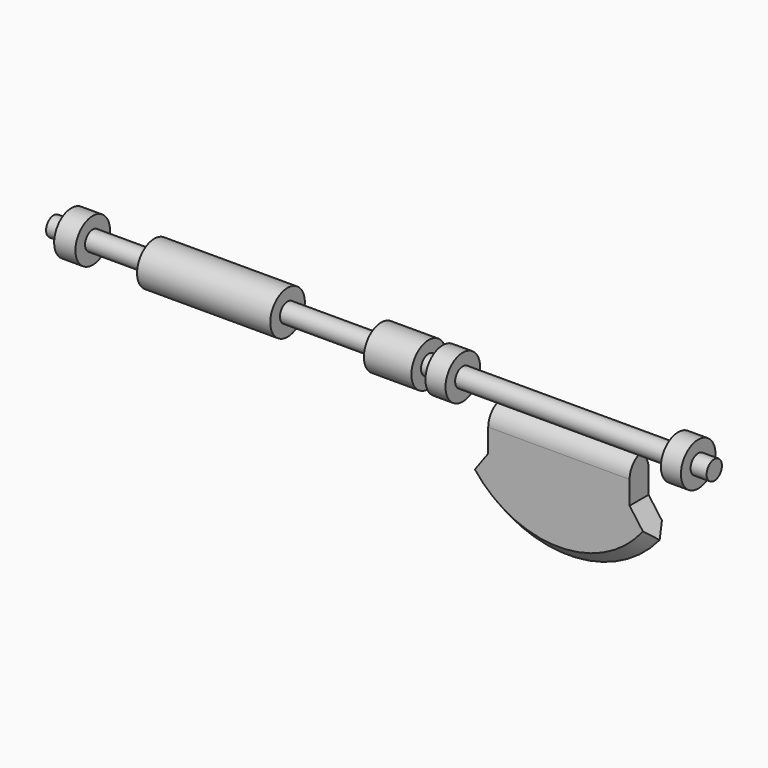
from build123d import *

# Parameters (mm, degrees)
F2_DEPTH    = 3.302
F3_DEPTH    = 3.302
F4_T2_ANGLE = 142.4839860816
F4_T4_ANGLE = 142.4839860816
F5_T1_DEPTH = 64.7221527338


# Not quite as in the source:
# - a fillet or chamfer that OpenCascade refuses, or shapes differently, is made with other operations: its cross-section is extruded or revolved along the edge and cut away or added


with BuildPart() as f1:
    # F0 (on Front) → F1 (revolve)
    with BuildSketch(Plane.XZ):
        Polygon((-57.3470704257, 12.4153448269), (-57.3470704257, 9.7549136262), (126.3579279184, 9.7549136262), (126.3579279184, 12.4153448269), (121.8937337399, 12.4153448269), (121.8937337399, 15.7655160874), (116.3134798408, 15.7655160874), (116.3134798408, 12.4153448269), (56.4188025892, 12.4153448269), (56.4188025892, 15.7655160874), (50.8385524154, 15.7655160874), (50.8385524154, 12.4153448269), (46.9323731959, 12.4153448269), (46.9323731959, 15.7655160874), (33.7257832289, 15.7655160874), (33.7257832289, 12.4153448269), (7.6856887899, 12.4153448269), (7.6856887899, 15.7655160874), (-29.3632764369, 15.7655160874), (-29.3632764369, 12.4153448269), (-46.5082786977, 12.4153448269), (-46.5082786977, 15.7655160874), (-52.420347929, 15.7655160874), (-52.420347929, 12.4153448269), align=None)
    revolve(axis=Axis((34.5054287463, 0, 9.7549136262), (1, 0, 0)))


with BuildPart() as f2:
    # F0 (on Front) → F2 (new body)
    with BuildSketch(Plane.XZ):
        with BuildLine():
            Line((105.4544225335, -4.4515635818), (105.4544225335, 7.0944824256))
            Line((105.4544225335, 7.0944824256), (66.1322697997, 7.0944824256))
            Line((66.1322697997, 7.0944824256), (66.1322697997, -4.4515635818))
            Line((66.1322697997, -4.4515635818), (59.3388823657, -13.8018592247))
            ThreePointArc((59.3388823657, -13.8018592247), (85.7933461666, -26.0433622806), (112.2478099675, -13.8018592247))
            Line((112.2478099675, -13.8018592247), (105.4544225335, -4.4515635818))
        make_face()
    extrude(amount=-F2_DEPTH)

    # F3 (add): a face of the model
    f3_faces = [f2.faces().sort_by_distance(p)[0] for p in [
        (85.7933461666, 0, -8.9000253062),
    ]]
    extrude(f3_faces, amount=F3_DEPTH)

    # F4: chamfer of 5.08 on 2 edges, made by hand

    # F4_s1 → F4_t2 (revolve, cut)
    with BuildSketch(Plane(origin=(6.2342301427, 0, -18.3570212695), x_dir=(0, 1, 0), z_dir=(-0.3215717936, 0, 0.9468851998))):
        Polygon((1.778, -49.3165019961), (-3.302, -54.3965019961), (-3.302, -49.3165019961), align=None)
    revolve(axis=Axis((85.7933461666, -3.302, 8.6620594386), (0, -1, 0)), revolution_arc=F4_T2_ANGLE, mode=Mode.SUBTRACT)

    # F4_s3 → F4_t4 (revolve, cut)
    with BuildSketch(Plane(origin=(6.2342301427, 0, -18.3570212695), x_dir=(0, 1, 0), z_dir=(-0.3215717936, 0, 0.9468851998))):
        Polygon((-1.778, -49.3165019961), (3.302, -54.3965019961), (3.302, -49.3165019961), align=None)
    revolve(axis=Axis((85.7933461666, 3.302, 8.6620594386), (0, -1, 0)), revolution_arc=F4_T4_ANGLE, mode=Mode.SUBTRACT)

    # F5: fillet of radius 5.08 on 2 edges, made by hand

    # F5_s2 → F5_t1 (cut)
    with BuildSketch(Plane.YZ.offset(53.4322697997)):
        with BuildLine():
            ThreePointArc((-3.302, 2.0144824256), (-1.8141024484, 5.606584874), (1.778, 7.0944824256))
            Line((1.778, 7.0944824256), (-3.302, 7.0944824256))
            Line((-3.302, 7.0944824256), (-3.302, 2.0144824256))
        make_face()
        with BuildLine():
            ThreePointArc((3.302, 2.0144824256), (1.8141024484, 5.606584874), (-1.778, 7.0944824256))
            Line((-1.778, 7.0944824256), (3.302, 7.0944824256))
            Line((3.302, 7.0944824256), (3.302, 2.0144824256))
        make_face()
    extrude(amount=F5_T1_DEPTH, mode=Mode.SUBTRACT)


solid = Compound([f1.part, f2.part])
